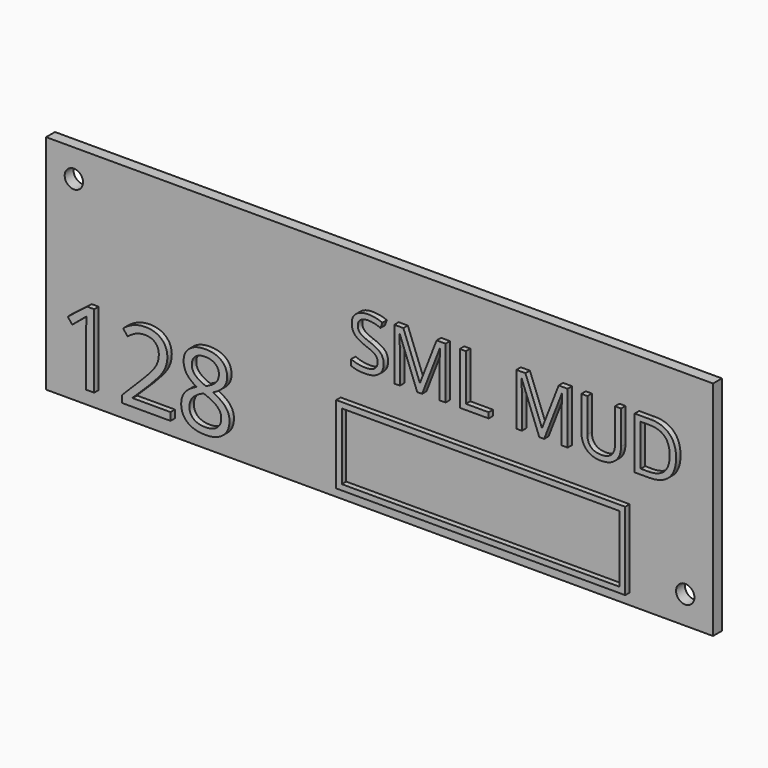
from build123d import *

# Parameters (mm, degrees)
F0_W         = 120
F0_H         = 40
F1_DEPTH     = 2
F3_D         = 3.3
F4_TEXT_SIZE = 13.0598918478
F5_DEPTH     = 1
F6_TEXT_SIZE = 18.5155049272
F7_DEPTH     = 1
F8_W         = 52
F8_H         = 14
F8_W_2       = 49.99999962
F8_H_2       = 11.99999962
F9_DEPTH     = 1


# Not quite as in the source:
# - Text() gives the source's letters only with a copy of the font that has no kerning and outlines rounded to 1/6400 em; it was checked with that copy


with BuildPart() as f1:
    # F0 (on Front) → F1 (new body)
    with BuildSketch(Plane.XZ):
        Rectangle(F0_W, F0_H)
    extrude(amount=F1_DEPTH)

    # F3 (through all)
    with Locations(Plane.XZ.offset(2)):
        with Locations((-55, 15), (55, -15)):
            Hole(F3_D / 2)

    # F4 (on face) → F5 (join)
    with BuildSketch(Plane.XZ.offset(2)):
        with Locations((-5, 2)):
            Text('SML MUD', F4_TEXT_SIZE, font='Open Sans', text_align=(TextAlign.LEFT, TextAlign.BOTTOM))
    extrude(amount=F5_DEPTH)

    # F6 (on face) → F7 (join)
    with BuildSketch(Plane.XZ.offset(2)):
        with Locations((-57, -17)):
            Text('128', F6_TEXT_SIZE, font='Open Sans', text_align=(TextAlign.LEFT, TextAlign.BOTTOM))
    extrude(amount=F7_DEPTH)

    # F8 (on face) → F9 (join)
    with BuildSketch(Plane.XZ.offset(2)):
        with Locations((19, -11)):
            Rectangle(F8_W, F8_H)
        with Locations((19, -11)):
            Rectangle(F8_W_2, F8_H_2, mode=Mode.SUBTRACT)
    extrude(amount=F9_DEPTH)


solid = f1.part
